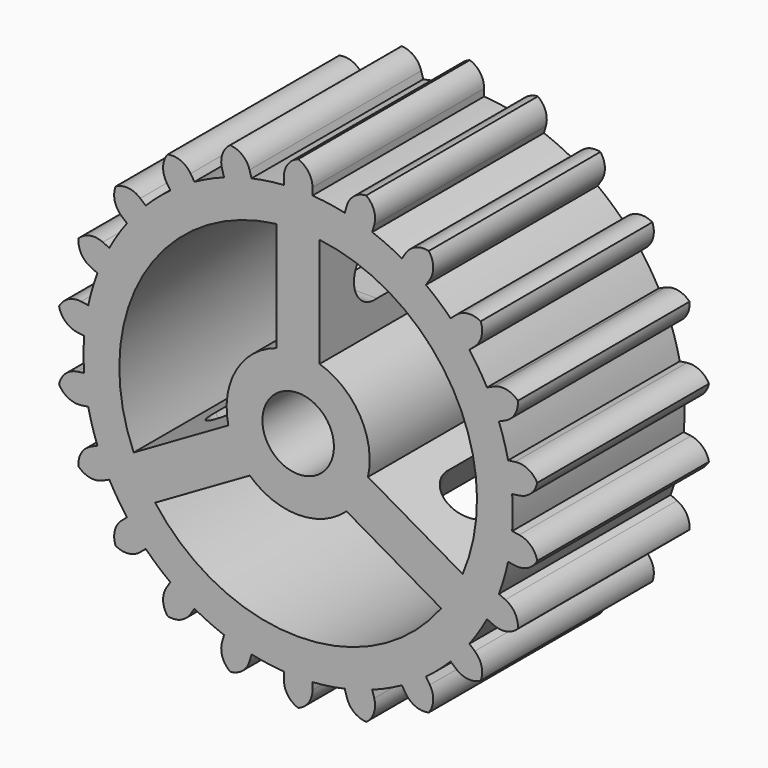
from build123d import *

# Parameters (mm, degrees)
F0_R        = 2.5
F1_DEPTH    = 15
F3_DEPTH    = 3
F5_DEPTH    = 3
F7_DEPTH    = 3
F8_T1_DEPTH = 22.5


# Not quite as in the source:
# - a fillet or chamfer that OpenCascade refuses, or shapes differently, is made with other operations: its cross-section is extruded or revolved along the edge and cut away or added


with BuildPart() as f1:
    # F0 (on Front) → F1 (new body)
    with BuildSketch(Plane.XZ):
        with BuildLine():
            Line((-1, 16.9666295471), (-1, 14.9666295471))
            ThreePointArc((-1, 14.9666295471), (-2.1347225741, 14.8473216282), (-3.257093836, 14.642108446))
            Line((-3.257093836, 14.642108446), (-3.8205589497, 16.5610943932))
            Line((-3.8205589497, 16.5610943932), (-5.7395448969, 15.9976292795))
            Line((-5.7395448969, 15.9976292795), (-5.1760797832, 14.0786433323))
            ThreePointArc((-5.1760797832, 14.0786433323), (-6.231225195, 13.6444799303), (-7.2503173001, 13.1313707985))
            Line((-7.2503173001, 13.1313707985), (-8.331598935, 14.8138778642))
            Line((-8.331598935, 14.8138778642), (-10.0141060006, 13.7325962293))
            Line((-10.0141060006, 13.7325962293), (-8.9328243657, 12.0500891636))
            ThreePointArc((-8.9328243657, 12.0500891636), (-9.8229110092, 11.3362436153), (-10.6561631758, 10.5568075843))
            Line((-10.6561631758, 10.5568075843), (-12.1676623245, 11.8665290521))
            Line((-12.1676623245, 11.8665290521), (-13.4773837924, 10.3550299034))
            Line((-13.4773837924, 10.3550299034), (-11.9658846437, 9.0453084355))
            ThreePointArc((-11.9658846437, 9.0453084355), (-12.6188029925, 8.1096122618), (-13.1987100857, 7.1269946033))
            Line((-13.1987100857, 7.1269946033), (-15.0179740764, 7.9578246293))
            Line((-15.0179740764, 7.9578246293), (-15.8488041024, 6.1385606386))
            Line((-15.8488041024, 6.1385606386), (-14.0295401117, 5.3077306125))
            ThreePointArc((-14.0295401117, 5.3077306125), (-14.3923946042, 4.2259883526), (-14.6719760001, 3.1197949054))
            Line((-14.6719760001, 3.1197949054), (-16.6516188839, 3.4044245819))
            Line((-16.6516188839, 3.4044245819), (-16.9362485604, 1.4247816982))
            Line((-16.9362485604, 1.4247816982), (-14.9566056767, 1.1401520216))
            ThreePointArc((-14.9566056767, 1.1401520216), (-15, 0), (-14.9566056767, -1.1401520216))
            Line((-14.9566056767, -1.1401520216), (-16.9362485604, -1.4247816982))
            Line((-16.9362485604, -1.4247816982), (-16.6516188839, -3.4044245819))
            Line((-16.6516188839, -3.4044245819), (-14.6719760001, -3.1197949054))
            ThreePointArc((-14.6719760001, -3.1197949054), (-14.3923946042, -4.2259883526), (-14.0295401117, -5.3077306125))
            Line((-14.0295401117, -5.3077306125), (-15.8488041024, -6.1385606386))
            Line((-15.8488041024, -6.1385606386), (-15.0179740764, -7.9578246293))
            Line((-15.0179740764, -7.9578246293), (-13.1987100857, -7.1269946033))
            ThreePointArc((-13.1987100857, -7.1269946033), (-12.6188029925, -8.1096122618), (-11.9658846437, -9.0453084355))
            Line((-11.9658846437, -9.0453084355), (-13.4773837924, -10.3550299034))
            Line((-13.4773837924, -10.3550299034), (-12.1676623245, -11.8665290521))
            Line((-12.1676623245, -11.8665290521), (-10.6561631758, -10.5568075843))
            ThreePointArc((-10.6561631758, -10.5568075843), (-9.8229110092, -11.3362436153), (-8.9328243657, -12.0500891636))
            Line((-8.9328243657, -12.0500891636), (-10.0141060006, -13.7325962293))
            Line((-10.0141060006, -13.7325962293), (-8.331598935, -14.8138778642))
            Line((-8.331598935, -14.8138778642), (-7.2503173001, -13.1313707985))
            ThreePointArc((-7.2503173001, -13.1313707985), (-6.231225195, -13.6444799303), (-5.1760797832, -14.0786433323))
            Line((-5.1760797832, -14.0786433323), (-5.7395448969, -15.9976292795))
            Line((-5.7395448969, -15.9976292795), (-3.8205589497, -16.5610943932))
            Line((-3.8205589497, -16.5610943932), (-3.257093836, -14.642108446))
            ThreePointArc((-3.257093836, -14.642108446), (-2.1347225741, -14.8473216282), (-1, -14.9666295471))
            Line((-1, -14.9666295471), (-1, -16.9666295471))
            Line((-1, -16.9666295471), (1, -16.9666295471))
            Line((1, -16.9666295471), (1, -14.9666295471))
            ThreePointArc((1, -14.9666295471), (2.1347225741, -14.8473216282), (3.257093836, -14.642108446))
            Line((3.257093836, -14.642108446), (3.8205589497, -16.5610943932))
            Line((3.8205589497, -16.5610943932), (5.7395448969, -15.9976292795))
            Line((5.7395448969, -15.9976292795), (5.1760797832, -14.0786433323))
            ThreePointArc((5.1760797832, -14.0786433323), (6.231225195, -13.6444799303), (7.2503173001, -13.1313707985))
            Line((7.2503173001, -13.1313707985), (8.331598935, -14.8138778642))
            Line((8.331598935, -14.8138778642), (10.0141060006, -13.7325962293))
            Line((10.0141060006, -13.7325962293), (8.9328243657, -12.0500891636))
            ThreePointArc((8.9328243657, -12.0500891636), (9.8229110092, -11.3362436153), (10.6561631758, -10.5568075843))
            Line((10.6561631758, -10.5568075843), (12.1676623245, -11.8665290521))
            Line((12.1676623245, -11.8665290521), (13.4773837924, -10.3550299034))
            Line((13.4773837924, -10.3550299034), (11.9658846437, -9.0453084355))
            ThreePointArc((11.9658846437, -9.0453084355), (12.6188029925, -8.1096122618), (13.1987100857, -7.1269946033))
            Line((13.1987100857, -7.1269946033), (15.0179740764, -7.9578246293))
            Line((15.0179740764, -7.9578246293), (15.8488041024, -6.1385606386))
            Line((15.8488041024, -6.1385606386), (14.0295401117, -5.3077306125))
            ThreePointArc((14.0295401117, -5.3077306125), (14.3923946042, -4.2259883526), (14.6719760001, -3.1197949054))
            Line((14.6719760001, -3.1197949054), (16.6516188839, -3.4044245819))
            Line((16.6516188839, -3.4044245819), (16.9362485604, -1.4247816982))
            Line((16.9362485604, -1.4247816982), (14.9566056767, -1.1401520216))
            ThreePointArc((14.9566056767, -1.1401520216), (15, 0), (14.9566056767, 1.1401520216))
            Line((14.9566056767, 1.1401520216), (16.9362485604, 1.4247816982))
            Line((16.9362485604, 1.4247816982), (16.6516188839, 3.4044245819))
            Line((16.6516188839, 3.4044245819), (14.6719760001, 3.1197949054))
            ThreePointArc((14.6719760001, 3.1197949054), (14.3923946042, 4.2259883526), (14.0295401117, 5.3077306125))
            Line((14.0295401117, 5.3077306125), (15.8488041024, 6.1385606386))
            Line((15.8488041024, 6.1385606386), (15.0179740764, 7.9578246293))
            Line((15.0179740764, 7.9578246293), (13.1987100857, 7.1269946033))
            ThreePointArc((13.1987100857, 7.1269946033), (12.6188029925, 8.1096122618), (11.9658846437, 9.0453084355))
            Line((11.9658846437, 9.0453084355), (13.4773837924, 10.3550299034))
            Line((13.4773837924, 10.3550299034), (12.1676623245, 11.8665290521))
            Line((12.1676623245, 11.8665290521), (10.6561631758, 10.5568075843))
            ThreePointArc((10.6561631758, 10.5568075843), (9.8229110092, 11.3362436153), (8.9328243657, 12.0500891636))
            Line((8.9328243657, 12.0500891636), (10.0141060006, 13.7325962293))
            Line((10.0141060006, 13.7325962293), (8.331598935, 14.8138778642))
            Line((8.331598935, 14.8138778642), (7.2503173001, 13.1313707985))
            ThreePointArc((7.2503173001, 13.1313707985), (6.231225195, 13.6444799303), (5.1760797832, 14.0786433323))
            Line((5.1760797832, 14.0786433323), (5.7395448969, 15.9976292795))
            Line((5.7395448969, 15.9976292795), (3.8205589497, 16.5610943932))
            Line((3.8205589497, 16.5610943932), (3.257093836, 14.642108446))
            ThreePointArc((3.257093836, 14.642108446), (2.1347225741, 14.8473216282), (1, 14.9666295471))
            Line((1, 14.9666295471), (1, 16.9666295471))
            Line((1, 16.9666295471), (-1, 16.9666295471))
        make_face()
        with BuildLine():
            Line((-9.9970926301, -7.5038749287), (-3.3806779105, -3.6838861092))
            ThreePointArc((-3.3806779105, -3.6838861092), (0, -5), (3.3806779105, -3.6838861092))
            Line((3.3806779105, -3.6838861092), (9.9970926301, -7.5038749287))
            ThreePointArc((9.9970926301, -7.5038749287), (0, -12.5), (-9.9970926301, -7.5038749287))
        make_face(mode=Mode.SUBTRACT)
        with BuildLine():
            ThreePointArc((-11.4970926301, -4.9057987173), (-10.8253175473, 6.25), (-1.5, 12.409673646))
            Line((-1.5, 12.409673646), (-1.5, 4.7696960071))
            ThreePointArc((-1.5, 4.7696960071), (-4.3301270189, 2.5), (-4.8806779105, -1.0858098979))
            Line((-4.8806779105, -1.0858098979), (-11.4970926301, -4.9057987173))
        make_face(mode=Mode.SUBTRACT)
        Circle(F0_R, mode=Mode.SUBTRACT)
        with BuildLine():
            Line((1.5, 4.7696960071), (1.5, 12.409673646))
            ThreePointArc((1.5, 12.409673646), (10.8253175473, 6.25), (11.4970926301, -4.9057987173))
            Line((11.4970926301, -4.9057987173), (4.8806779105, -1.0858098979))
            ThreePointArc((4.8806779105, -1.0858098979), (4.3301270189, 2.5), (1.5, 4.7696960071))
        make_face(mode=Mode.SUBTRACT)
    extrude(amount=F1_DEPTH)

    # F2 (on face) → F3 (cut, through all)
    with BuildSketch(Plane(origin=(0.75, 0, 1.2990381057), x_dir=(0.8660254038, 0, -0.5), z_dir=(0.5, 0, 0.8660254038))):
        with BuildLine():
            Line((6.7696960071, -5), (6.7696960071, -10))
            ThreePointArc((6.7696960071, -10), (8.5896848265, -12), (10.409673646, -10))
            Line((10.409673646, -10), (10.409673646, -5))
            ThreePointArc((10.409673646, -5), (8.5896848265, -3), (6.7696960071, -5))
        make_face()
    extrude(amount=-F3_DEPTH, mode=Mode.SUBTRACT)

    # F4 (on face) → F5 (cut, through all)
    with BuildSketch(Plane(origin=(-0.75, 0, 1.2990381057), x_dir=(0.8660254038, 0, 0.5), z_dir=(-0.5, 0, 0.8660254038))):
        with BuildLine():
            Line((-10.409673646, -5), (-10.409673646, -10))
            ThreePointArc((-10.409673646, -10), (-8.5896848265, -12), (-6.7696960071, -10))
            Line((-6.7696960071, -10), (-6.7696960071, -5))
            ThreePointArc((-6.7696960071, -5), (-8.5896848265, -3), (-10.409673646, -5))
        make_face()
    extrude(amount=-F5_DEPTH, mode=Mode.SUBTRACT)

    # F6 (on face) → F7 (cut, through all)
    with BuildSketch(Plane(origin=(-1.5, 0, 0), x_dir=(0, -1, 0), z_dir=(-1, 0, 0))):
        with BuildLine():
            Line((10, 10.409673646), (5, 10.409673646))
            ThreePointArc((5, 10.409673646), (3, 8.5896848265), (5, 6.7696960071))
            Line((5, 6.7696960071), (10, 6.7696960071))
            ThreePointArc((10, 6.7696960071), (12, 8.5896848265), (10, 10.409673646))
        make_face()
    extrude(amount=-F7_DEPTH, mode=Mode.SUBTRACT)

    # F8: fillet of radius 1.5 on 44 edges, made by hand

    # F8_s2 → F8_t1 (cut)
    with BuildSketch(Plane.XZ.offset(-3.75)):
        with BuildLine():
            ThreePointArc((-13.1499534254, -10.7329046906), (-12.1233378387, -11.2467917616), (-11.034037963, -10.8842379512))
            Line((-11.034037963, -10.8842379512), (-12.1676623245, -11.8665290521))
            Line((-12.1676623245, -11.8665290521), (-13.1499534254, -10.7329046906))
        make_face()
        with BuildLine():
            ThreePointArc((-12.3437594309, -9.3727388025), (-12.8576465019, -10.3993543892), (-12.4950926915, -11.488654265))
            Line((-12.4950926915, -11.488654265), (-13.4773837924, -10.3550299034))
            Line((-13.4773837924, -10.3550299034), (-12.3437594309, -9.3727388025))
        make_face()
        with BuildLine():
            ThreePointArc((-15.6410965959, -6.5933766362), (-14.8008448722, -7.3756787042), (-13.6535260833, -7.3347021098))
            Line((-13.6535260833, -7.3347021098), (-15.0179740764, -7.9578246293))
            Line((-15.0179740764, -7.9578246293), (-15.6410965959, -6.5933766362))
        make_face()
        with BuildLine():
            ThreePointArc((-14.4843561093, -5.515438119), (-15.2666581773, -6.3556898427), (-15.2256815829, -7.5030086316))
            Line((-15.2256815829, -7.5030086316), (-15.8488041024, -6.1385606386))
            Line((-15.8488041024, -6.1385606386), (-14.4843561093, -5.515438119))
        make_face()
        with BuildLine():
            ThreePointArc((-15.4515163976, -1.2113094407), (-16.4388560016, -1.7971251038), (-16.722776303, -2.909513861))
            Line((-16.722776303, -2.909513861), (-16.9362485604, -1.4247816982))
            Line((-16.9362485604, -1.4247816982), (-15.4515163976, -1.2113094407))
        make_face()
        with BuildLine():
            ThreePointArc((-16.8650911413, -1.9196924191), (-16.2792754782, -2.9070320231), (-15.1668867211, -3.1909523245))
            Line((-15.1668867211, -3.1909523245), (-16.6516188839, -3.4044245819))
            Line((-16.6516188839, -3.4044245819), (-16.8650911413, -1.9196924191))
        make_face()
        with BuildLine():
            ThreePointArc((-15.1668867211, 3.1909523245), (-16.2792754782, 2.9070320231), (-16.8650911413, 1.9196924191))
            Line((-16.8650911413, 1.9196924191), (-16.6516188839, 3.4044245819))
            Line((-16.6516188839, 3.4044245819), (-15.1668867211, 3.1909523245))
        make_face()
        with BuildLine():
            ThreePointArc((-16.722776303, 2.909513861), (-16.4388560016, 1.7971251038), (-15.4515163976, 1.2113094407))
            Line((-15.4515163976, 1.2113094407), (-16.9362485604, 1.4247816982))
            Line((-16.9362485604, 1.4247816982), (-16.722776303, 2.909513861))
        make_face()
        with BuildLine():
            ThreePointArc((-13.6535260833, 7.3347021098), (-14.8008448722, 7.3756787042), (-15.6410965959, 6.5933766362))
            Line((-15.6410965959, 6.5933766362), (-15.0179740764, 7.9578246293))
            Line((-15.0179740764, 7.9578246293), (-13.6535260833, 7.3347021098))
        make_face()
        with BuildLine():
            ThreePointArc((-15.2256815829, 7.5030086316), (-15.2666581773, 6.3556898427), (-14.4843561093, 5.515438119))
            Line((-14.4843561093, 5.515438119), (-15.8488041024, 6.1385606386))
            Line((-15.8488041024, 6.1385606386), (-15.2256815829, 7.5030086316))
        make_face()
        with BuildLine():
            ThreePointArc((-11.034037963, 10.8842379512), (-12.1233378387, 11.2467917616), (-13.1499534254, 10.7329046906))
            Line((-13.1499534254, 10.7329046906), (-12.1676623245, 11.8665290521))
            Line((-12.1676623245, 11.8665290521), (-11.034037963, 10.8842379512))
        make_face()
        with BuildLine():
            ThreePointArc((-12.4950926915, 11.488654265), (-12.8576465019, 10.3993543892), (-12.3437594309, 9.3727388025))
            Line((-12.3437594309, 9.3727388025), (-13.4773837924, 10.3550299034))
            Line((-13.4773837924, 10.3550299034), (-12.4950926915, 11.488654265))
        make_face()
        with BuildLine():
            ThreePointArc((-7.5206377088, 13.5519975649), (-8.4636700737, 14.2067566377), (-9.5934792342, 14.002916638))
            Line((-9.5934792342, 14.002916638), (-8.331598935, 14.8138778642))
            Line((-8.331598935, 14.8138778642), (-7.5206377088, 13.5519975649))
        make_face()
        with BuildLine():
            ThreePointArc((-8.7522257014, 14.5435574555), (-9.4069847742, 13.6005250905), (-9.2031447745, 12.47071593))
            Line((-9.2031447745, 12.47071593), (-10.0141060006, 13.7325962293))
            Line((-10.0141060006, 13.7325962293), (-8.7522257014, 14.5435574555))
        make_face()
        with BuildLine():
            ThreePointArc((-4.3003054365, 16.4202281148), (-5.1942250856, 15.6998621344), (-5.3169460616, 14.5583898191))
            Line((-5.3169460616, 14.5583898191), (-5.7395448969, 15.9976292795))
            Line((-5.7395448969, 15.9976292795), (-4.3003054365, 16.4202281148))
        make_face()
        with BuildLine():
            ThreePointArc((-3.3979601144, 15.1218549328), (-4.1183260947, 16.0157745819), (-5.2597984101, 16.1384955579))
            Line((-5.2597984101, 16.1384955579), (-3.8205589497, 16.5610943932))
            Line((-3.8205589497, 16.5610943932), (-3.3979601144, 15.1218549328))
        make_face()
        with BuildLine():
            ThreePointArc((0.5, 16.9666295471), (-0.5606601718, 16.5272897189), (-1, 15.4666295471))
            Line((-1, 15.4666295471), (-1, 16.9666295471))
            Line((-1, 16.9666295471), (0.5, 16.9666295471))
        make_face()
        with BuildLine():
            ThreePointArc((1, 15.4666295471), (0.5606601718, 16.5272897189), (-0.5, 16.9666295471))
            Line((-0.5, 16.9666295471), (1, 16.9666295471))
            Line((1, 16.9666295471), (1, 15.4666295471))
        make_face()
        with BuildLine():
            ThreePointArc((5.2597984101, 16.1384955579), (4.1183260947, 16.0157745819), (3.3979601144, 15.1218549328))
            Line((3.3979601144, 15.1218549328), (3.8205589497, 16.5610943932))
            Line((3.8205589497, 16.5610943932), (5.2597984101, 16.1384955579))
        make_face()
        with BuildLine():
            ThreePointArc((5.3169460616, 14.5583898191), (5.1942250856, 15.6998621344), (4.3003054365, 16.4202281148))
            Line((4.3003054365, 16.4202281148), (5.7395448969, 15.9976292795))
            Line((5.7395448969, 15.9976292795), (5.3169460616, 14.5583898191))
        make_face()
        with BuildLine():
            ThreePointArc((7.5206377088, 13.5519975649), (8.4636700737, 14.2067566377), (9.5934792342, 14.002916638))
            Line((9.5934792342, 14.002916638), (8.331598935, 14.8138778642))
            Line((8.331598935, 14.8138778642), (7.5206377088, 13.5519975649))
        make_face()
        with BuildLine():
            ThreePointArc((8.7522257014, 14.5435574555), (9.4069847742, 13.6005250905), (9.2031447745, 12.47071593))
            Line((9.2031447745, 12.47071593), (10.0141060006, 13.7325962293))
            Line((10.0141060006, 13.7325962293), (8.7522257014, 14.5435574555))
        make_face()
        with BuildLine():
            ThreePointArc((13.1499534254, 10.7329046906), (12.1233378387, 11.2467917616), (11.034037963, 10.8842379512))
            Line((11.034037963, 10.8842379512), (12.1676623245, 11.8665290521))
            Line((12.1676623245, 11.8665290521), (13.1499534254, 10.7329046906))
        make_face()
        with BuildLine():
            ThreePointArc((12.3437594309, 9.3727388025), (12.8576465019, 10.3993543892), (12.4950926915, 11.488654265))
            Line((12.4950926915, 11.488654265), (13.4773837924, 10.3550299034))
            Line((13.4773837924, 10.3550299034), (12.3437594309, 9.3727388025))
        make_face()
        with BuildLine():
            ThreePointArc((14.4843561093, 5.515438119), (15.2666581773, 6.3556898427), (15.2256815829, 7.5030086316))
            Line((15.2256815829, 7.5030086316), (15.8488041024, 6.1385606386))
            Line((15.8488041024, 6.1385606386), (14.4843561093, 5.515438119))
        make_face()
        with BuildLine():
            ThreePointArc((15.6410965959, 6.5933766362), (14.8008448722, 7.3756787042), (13.6535260833, 7.3347021098))
            Line((13.6535260833, 7.3347021098), (15.0179740764, 7.9578246293))
            Line((15.0179740764, 7.9578246293), (15.6410965959, 6.5933766362))
        make_face()
        with BuildLine():
            ThreePointArc((15.4515163976, 1.2113094407), (16.4388560016, 1.7971251038), (16.722776303, 2.909513861))
            Line((16.722776303, 2.909513861), (16.9362485604, 1.4247816982))
            Line((16.9362485604, 1.4247816982), (15.4515163976, 1.2113094407))
        make_face()
        with BuildLine():
            ThreePointArc((16.8650911413, 1.9196924191), (16.2792754782, 2.9070320231), (15.1668867211, 3.1909523245))
            Line((15.1668867211, 3.1909523245), (16.6516188839, 3.4044245819))
            Line((16.6516188839, 3.4044245819), (16.8650911413, 1.9196924191))
        make_face()
        with BuildLine():
            ThreePointArc((15.1668867211, -3.1909523245), (16.2792754782, -2.9070320231), (16.8650911413, -1.9196924191))
            Line((16.8650911413, -1.9196924191), (16.6516188839, -3.4044245819))
            Line((16.6516188839, -3.4044245819), (15.1668867211, -3.1909523245))
        make_face()
        with BuildLine():
            ThreePointArc((16.722776303, -2.909513861), (16.4388560016, -1.7971251038), (15.4515163976, -1.2113094407))
            Line((15.4515163976, -1.2113094407), (16.9362485604, -1.4247816982))
            Line((16.9362485604, -1.4247816982), (16.722776303, -2.909513861))
        make_face()
        with BuildLine():
            ThreePointArc((15.2256815829, -7.5030086316), (15.2666581773, -6.3556898427), (14.4843561093, -5.515438119))
            Line((14.4843561093, -5.515438119), (15.8488041024, -6.1385606386))
            Line((15.8488041024, -6.1385606386), (15.2256815829, -7.5030086316))
        make_face()
        with BuildLine():
            ThreePointArc((13.6535260833, -7.3347021098), (14.8008448722, -7.3756787042), (15.6410965959, -6.5933766362))
            Line((15.6410965959, -6.5933766362), (15.0179740764, -7.9578246293))
            Line((15.0179740764, -7.9578246293), (13.6535260833, -7.3347021098))
        make_face()
        with BuildLine():
            ThreePointArc((12.4950926915, -11.488654265), (12.8576465019, -10.3993543892), (12.3437594309, -9.3727388025))
            Line((12.3437594309, -9.3727388025), (13.4773837924, -10.3550299034))
            Line((13.4773837924, -10.3550299034), (12.4950926915, -11.488654265))
        make_face()
        with BuildLine():
            ThreePointArc((11.034037963, -10.8842379512), (12.1233378387, -11.2467917616), (13.1499534254, -10.7329046906))
            Line((13.1499534254, -10.7329046906), (12.1676623245, -11.8665290521))
            Line((12.1676623245, -11.8665290521), (11.034037963, -10.8842379512))
        make_face()
        with BuildLine():
            ThreePointArc((8.7522257014, -14.5435574555), (9.4069847742, -13.6005250905), (9.2031447745, -12.47071593))
            Line((9.2031447745, -12.47071593), (10.0141060006, -13.7325962293))
            Line((10.0141060006, -13.7325962293), (8.7522257014, -14.5435574555))
        make_face()
        with BuildLine():
            ThreePointArc((7.5206377088, -13.5519975649), (8.4636700737, -14.2067566377), (9.5934792342, -14.002916638))
            Line((9.5934792342, -14.002916638), (8.331598935, -14.8138778642))
            Line((8.331598935, -14.8138778642), (7.5206377088, -13.5519975649))
        make_face()
        with BuildLine():
            ThreePointArc((4.3003054365, -16.4202281148), (5.1942250856, -15.6998621344), (5.3169460616, -14.5583898191))
            Line((5.3169460616, -14.5583898191), (5.7395448969, -15.9976292795))
            Line((5.7395448969, -15.9976292795), (4.3003054365, -16.4202281148))
        make_face()
        with BuildLine():
            ThreePointArc((3.3979601144, -15.1218549328), (4.1183260947, -16.0157745819), (5.2597984101, -16.1384955579))
            Line((5.2597984101, -16.1384955579), (3.8205589497, -16.5610943932))
            Line((3.8205589497, -16.5610943932), (3.3979601144, -15.1218549328))
        make_face()
        with BuildLine():
            ThreePointArc((-0.5, -16.9666295471), (0.5606601718, -16.5272897189), (1, -15.4666295471))
            Line((1, -15.4666295471), (1, -16.9666295471))
            Line((1, -16.9666295471), (-0.5, -16.9666295471))
        make_face()
        with BuildLine():
            ThreePointArc((-1, -15.4666295471), (-0.5606601718, -16.5272897189), (0.5, -16.9666295471))
            Line((0.5, -16.9666295471), (-1, -16.9666295471))
            Line((-1, -16.9666295471), (-1, -15.4666295471))
        make_face()
        with BuildLine():
            ThreePointArc((-5.2597984101, -16.1384955579), (-4.1183260947, -16.0157745819), (-3.3979601144, -15.1218549328))
            Line((-3.3979601144, -15.1218549328), (-3.8205589497, -16.5610943932))
            Line((-3.8205589497, -16.5610943932), (-5.2597984101, -16.1384955579))
        make_face()
        with BuildLine():
            ThreePointArc((-5.3169460616, -14.5583898191), (-5.1942250856, -15.6998621344), (-4.3003054365, -16.4202281148))
            Line((-4.3003054365, -16.4202281148), (-5.7395448969, -15.9976292795))
            Line((-5.7395448969, -15.9976292795), (-5.3169460616, -14.5583898191))
        make_face()
        with BuildLine():
            ThreePointArc((-9.5934792342, -14.002916638), (-8.4636700737, -14.2067566377), (-7.5206377088, -13.5519975649))
            Line((-7.5206377088, -13.5519975649), (-8.331598935, -14.8138778642))
            Line((-8.331598935, -14.8138778642), (-9.5934792342, -14.002916638))
        make_face()
        with BuildLine():
            ThreePointArc((-9.2031447745, -12.47071593), (-9.4069847742, -13.6005250905), (-8.7522257014, -14.5435574555))
            Line((-8.7522257014, -14.5435574555), (-10.0141060006, -13.7325962293))
            Line((-10.0141060006, -13.7325962293), (-9.2031447745, -12.47071593))
        make_face()
    extrude(amount=F8_T1_DEPTH, mode=Mode.SUBTRACT)


solid = f1.part
